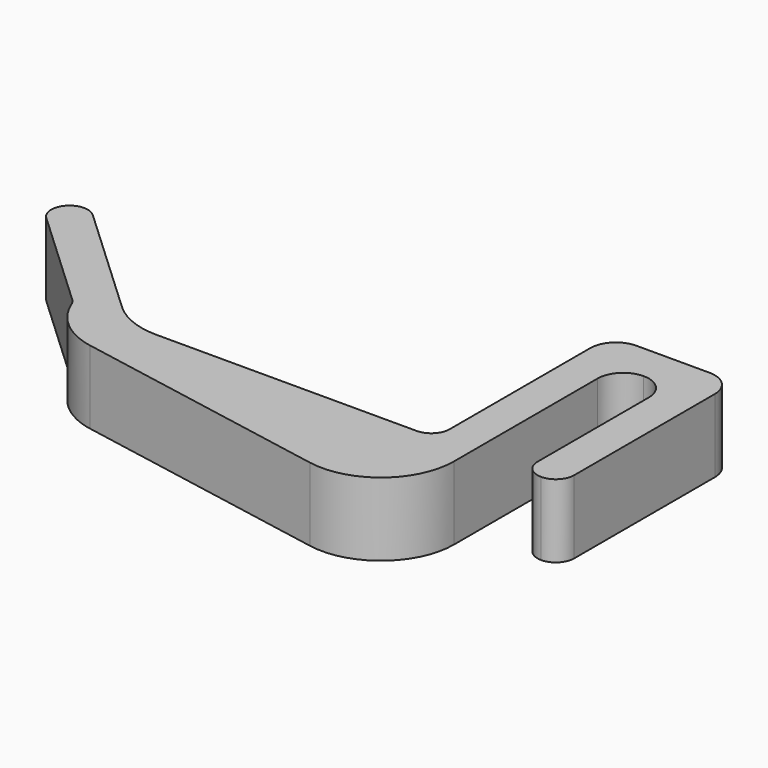
from build123d import *

# Parameters (mm, degrees)
F1_DEPTH = 10
F2_R     = 3.49999
F3_R     = 2.49999
F4_R     = 10


# Not quite as in the source:
# - a fillet or chamfer is up to 0.001 mm smaller than in the source, because OpenCascade refuses the exact size


with BuildPart() as f1:
    # F0 (on Top) → F1 (new body)
    with BuildSketch(Plane.XY):
        Polygon((5, -15), (5, 0), (5, 25), (12, 25), (12, 0), (17, 0), (17, 30), (0, 30), (0, 0), (-42, 0), (-49.3313959282, 0), (-49.3313959282, -5), align=None)
        Polygon((-65.8878954456, 15.4391855737), (-49.3313959282, 0), (-42, 0), (-62.4779036453, 19.0959540817), align=None)
    extrude(amount=F1_DEPTH)

    # F2 (radius 3.5 in the source; OpenCascade refuses exactly that, so slightly less here)
    f2_edges = [f1.edges().sort_by_distance(p)[0] for p in [
        (5, 25, 5),
        (12, 25, 5),
        (0, 30, 5),
        (17, 30, 5),
    ]]
    fillet(f2_edges, radius=F2_R)

    # F3 (radius 2.5 in the source; OpenCascade refuses exactly that, so slightly less here)
    f3_edges = [f1.edges().sort_by_distance(p)[0] for p in [
        (0, 0, 5),
        (17, 0, 5),
        (12, 0, 5),
        (-49.331396, 0, 5),
        (-62.477904, 19.095954, 5),
        (-65.887895, 15.439186, 5),
    ]]
    fillet(f3_edges, radius=F3_R)

    # F4
    f4_edges = [f1.edges().sort_by_distance(p)[0] for p in [
        (-2.49999, 0, 5),
        (5, -15, 5),
        (-49.331396, -5, 5),
        (-42, 0, 5),
    ]]
    fillet(f4_edges, radius=F4_R)


solid = f1.part
